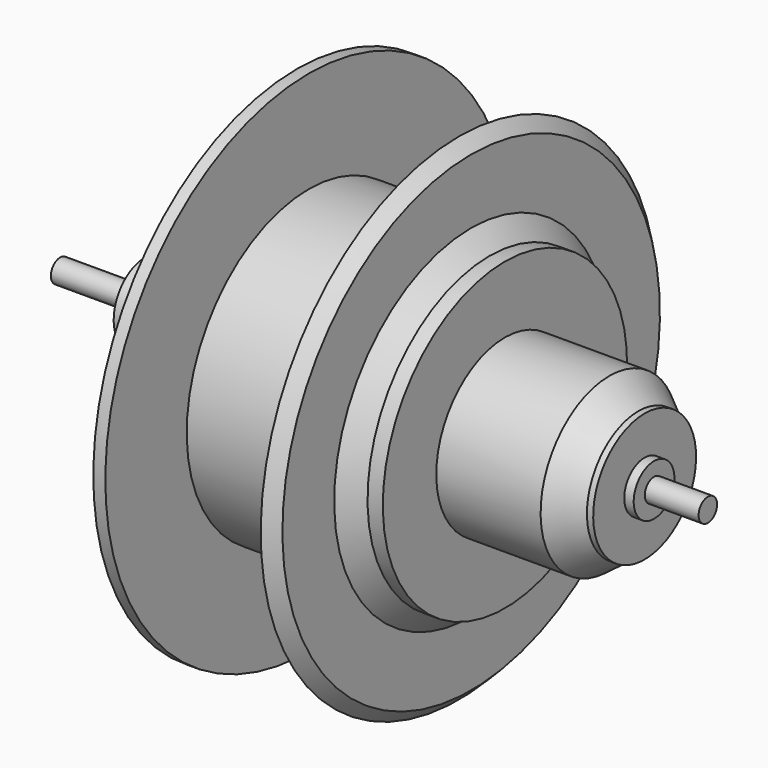
from build123d import *

# Parameters (mm, degrees)
F0_R     = 3.175
F1_DEPTH = 88.9


# Not quite as in the source:
# - a fillet or chamfer that OpenCascade refuses, or shapes differently, is made with other operations: its cross-section is extruded or revolved along the edge and cut away or added


with BuildPart() as f1:
    # F0 (on Right) → F1 (new body, symmetric)
    with BuildSketch(Plane.YZ):
        Circle(F0_R)
    extrude(amount=F1_DEPTH, both=True)


with BuildPart() as f3:
    # F2 (on Front) → F3 (revolve)
    with BuildSketch(Plane.XZ):
        Polygon((-65.5721798539, 10.789279826), (-65.5721798539, 3.175), (74.1278201461, 3.175), (74.1278201461, 6.985), (71.5452923138, 6.985), (71.5452923138, 17.653), (69.8267191484, 17.653), (61.8413901258, 23.561832648), (33.2043394446, 23.561832648), (33.2043394446, 41.91), (23.9228336141, 41.91), (23.9228336141, 69.85), (20.6208336141, 69.85), (20.6208336141, 41.91), (-20.6208336141, 41.91), (-20.6208336141, 69.85), (-23.9228336141, 69.85), (-23.9228336141, 41.91), (-33.2043394446, 41.91), (-33.2043394446, 20.32), (-36.4167802036, 20.32), (-37.4993234873, 19.685), (-43.0255383253, 19.685), (-43.0255383253, 10.789279826), align=None)
    revolve(axis=Axis((54.40691486, 0, 0), (1, 0, 0)))

    # F5: chamfer of 5.08 on 2 edges, made by hand

    # F5_s1 → F5_t2 (revolve)
    with BuildSketch(Plane.XZ):
        Polygon((29.0028336141, 41.91), (23.9228336141, 46.99), (23.9228336141, 41.91), align=None)
    revolve(axis=Axis((23.9228336141, 0, 0), (1, 0, 0)))

    # F5_s3 → F5_t4 (revolve, cut)
    with BuildSketch(Plane.XZ):
        Polygon((23.9228336141, 64.77), (18.8428336141, 69.85), (23.9228336141, 69.85), align=None)
    revolve(axis=Axis((23.9228336141, 0, 0), (1, 0, 0)), mode=Mode.SUBTRACT)


solid = Compound([f1.part, f3.part])
